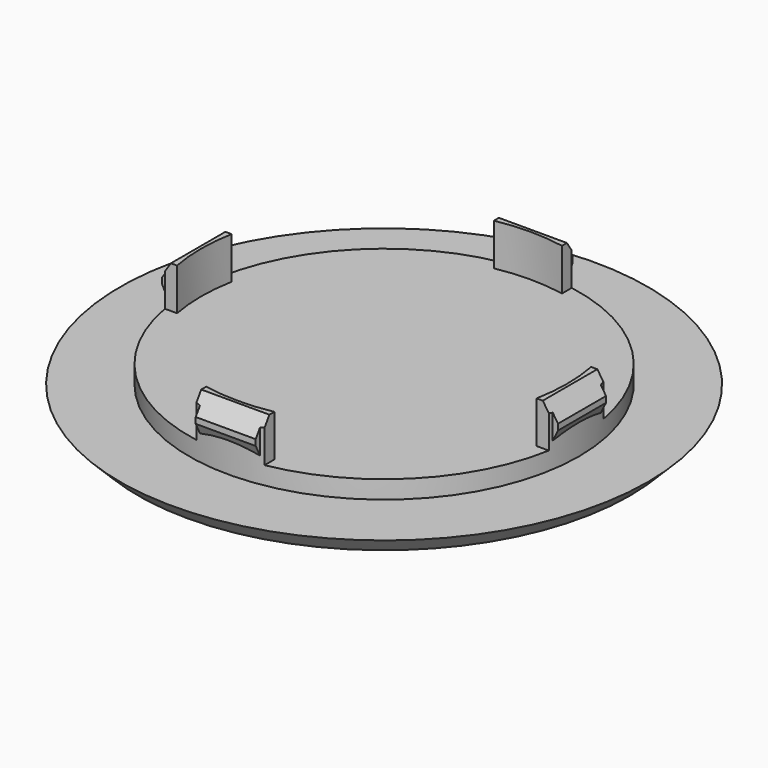
from build123d import *

# Parameters (mm, degrees)
F0_R          = 41
F1_DEPTH      = 3
F1_TAPER      = -45
F2_R          = 32.5
F3_DEPTH      = 10
F4_W          = 10
F4_H          = 6
F6_DEPTH      = 33
F6_DEPTH_BACK = 33
F7_W          = 10
F7_H          = 6
F8_DEPTH      = 33
F8_DEPTH_BACK = 33
F5_R          = 30.5
F9_DEPTH      = 7
F12_DEPTH     = 7
F13_SIZE2     = 2
F13_SIZE      = 3
F13_2_SIZE2   = 2
F13_2_SIZE    = 3
F14_SIZE2     = 3
F14_SIZE      = 2
F14_2_SIZE2   = 3
F14_2_SIZE    = 2
F15_T4_DEPTH  = 20.3593154951
F15_S5_R      = 32.5
F15_T6_DEPTH  = 12
F15_T10_DEPTH = 20.3593154951
F15_S11_R     = 32.5
F15_T12_DEPTH = 12
F16_T4_DEPTH  = 20.3593154951
F16_S5_R      = 32.5
F16_T6_DEPTH  = 12
F16_T10_DEPTH = 20.3593154951
F16_S11_R     = 32.5
F16_T12_DEPTH = 12


# Not quite as in the source:
# - a fillet or chamfer that OpenCascade refuses, or shapes differently, is made with other operations: its cross-section is extruded or revolved along the edge and cut away or added


with BuildPart() as f1:
    # F0 (on Top) → F1 (new body)
    with BuildSketch(Plane.XY):
        Circle(F0_R)
    extrude(amount=F1_DEPTH, taper=F1_TAPER)

    # F2 (on face) → F3 (join)
    with BuildSketch(Plane.XY.offset(3)):
        Circle(F2_R)
    extrude(amount=F3_DEPTH)

    # F4 (on Front) → F6 (join, two sides)
    with BuildSketch(Plane.XZ) as f6_sk:
        with Locations((0, 10)):
            Rectangle(F4_W, F4_H)
    extrude(amount=F6_DEPTH)
    extrude(f6_sk.sketch, amount=-F6_DEPTH_BACK)

    # F7 (on Right) → F8 (join, two sides)
    with BuildSketch(Plane.YZ) as f8_sk:
        with Locations((0, 10)):
            Rectangle(F7_W, F7_H)
    extrude(amount=F8_DEPTH)
    extrude(f8_sk.sketch, amount=-F8_DEPTH_BACK)

    # F5 (on face) → F9 (cut)
    with BuildSketch(Plane.XY.offset(13)):
        Circle(F5_R)
    extrude(amount=-F9_DEPTH, mode=Mode.SUBTRACT)

    # F11 (on face) → F12 (cut)
    with BuildSketch(Plane.XY.offset(13)):
        with BuildLine():
            ThreePointArc((-5.6789083458, 32), (-22.9809703886, 22.9809703886), (-32, 5.6789083458))
            Line((-32, 5.6789083458), (-29.9666481275, 5.6789083458))
            ThreePointArc((-29.9666481275, 5.6789083458), (-21.5667568262, 21.5667568262), (-5.6789083458, 29.9666481275))
            Line((-5.6789083458, 29.9666481275), (-5.6789083458, 32))
        make_face()
        with BuildLine():
            ThreePointArc((-5.6789083458, 29.9666481275), (-21.5667568262, 21.5667568262), (-29.9666481275, 5.6789083458))
            ThreePointArc((-29.9666481275, 5.6789083458), (-30.5, 0), (-29.9666481275, -5.6789083458))
            ThreePointArc((-29.9666481275, -5.6789083458), (-21.5667568262, -21.5667568262), (-5.6789083458, -29.9666481275))
            ThreePointArc((-5.6789083458, -29.9666481275), (0, -30.5), (5.6789083458, -29.9666481275))
            ThreePointArc((5.6789083458, -29.9666481275), (21.5667568262, -21.5667568262), (29.9666481275, -5.6789083458))
            ThreePointArc((29.9666481275, -5.6789083458), (30.3663692915, -2.8519495183), (30.5, 0))
            ThreePointArc((30.5, 0), (30.3663692915, 2.8519495183), (29.9666481275, 5.6789083458))
            ThreePointArc((29.9666481275, 5.6789083458), (21.5667568262, 21.5667568262), (5.6789083458, 29.9666481275))
            ThreePointArc((5.6789083458, 29.9666481275), (0, 30.5), (-5.6789083458, 29.9666481275))
        make_face()
        with BuildLine():
            Line((5.6789083458, 32), (5.6789083458, 29.9666481275))
            ThreePointArc((5.6789083458, 29.9666481275), (21.5667568262, 21.5667568262), (29.9666481275, 5.6789083458))
            Line((29.9666481275, 5.6789083458), (32, 5.6789083458))
            ThreePointArc((32, 5.6789083458), (22.9809703886, 22.9809703886), (5.6789083458, 32))
        make_face()
        with BuildLine():
            ThreePointArc((29.9666481275, -5.6789083458), (21.5667568262, -21.5667568262), (5.6789083458, -29.9666481275))
            Line((5.6789083458, -29.9666481275), (5.6789083458, -32))
            ThreePointArc((5.6789083458, -32), (22.9809703886, -22.9809703886), (32, -5.6789083458))
            Line((32, -5.6789083458), (29.9666481275, -5.6789083458))
        make_face()
        with BuildLine():
            ThreePointArc((-5.6789083458, -29.9666481275), (-21.5667568262, -21.5667568262), (-29.9666481275, -5.6789083458))
            Line((-29.9666481275, -5.6789083458), (-32, -5.6789083458))
            ThreePointArc((-32, -5.6789083458), (-22.9809703886, -22.9809703886), (-5.6789083458, -32))
            Line((-5.6789083458, -32), (-5.6789083458, -29.9666481275))
        make_face()
    extrude(amount=-F12_DEPTH, mode=Mode.SUBTRACT)

    # F13
    f13_edges = [f1.edges().sort_by_distance(p)[0] for p in [
        (0, 33, 13),
    ]]
    f13_side = f1.faces().sort_by_distance((0, 33, 10))[0]
    chamfer(f13_edges, length=F13_SIZE, length2=F13_SIZE2, reference=f13_side)

    # F13#2
    f13_2_edges = [f1.edges().sort_by_distance(p)[0] for p in [
        (33, 0, 13),
    ]]
    f13_2_side = f1.faces().sort_by_distance((33, 0, 10))[0]
    chamfer(f13_2_edges, length=F13_2_SIZE, length2=F13_2_SIZE2, reference=f13_2_side)

    # F14
    f14_edges = [f1.edges().sort_by_distance(p)[0] for p in [
        (0, -33, 13),
    ]]
    f14_side = f1.faces().sort_by_distance((0, -31.618427, 13))[0]
    chamfer(f14_edges, length=F14_SIZE, length2=F14_SIZE2, reference=f14_side)

    # F14#2
    f14_2_edges = [f1.edges().sort_by_distance(p)[0] for p in [
        (-33, 0, 13),
    ]]
    f14_2_side = f1.faces().sort_by_distance((-31.618427, 0, 13))[0]
    chamfer(f14_2_edges, length=F14_2_SIZE, length2=F14_2_SIZE2, reference=f14_2_side)

    # F15: chamfer of 1 x 2 on 2 edges, made by hand


with BuildPart() as f15_tool2:
    # F15_s3 → F15_t4 (new body)
    with BuildSketch(Plane.XZ.offset(10.1796577476)):
        Polygon((32, 7), (33, 9), (33, 7), align=None)
    extrude(amount=-F15_T4_DEPTH)

    # F15_s5 → F15_t6 (cut, symmetric)
    with BuildSketch(Plane.XY.offset(8)):
        Circle(F15_S5_R)
    extrude(amount=F15_T6_DEPTH, both=True, mode=Mode.SUBTRACT)


with BuildPart() as f1_1:
    add(f1.part)

    # F15_t1: cut F15_tool2
    add(f15_tool2.part, mode=Mode.SUBTRACT)


with BuildPart() as f15_tool8:
    # F15_s9 → F15_t10 (new body)
    with BuildSketch(Plane.YZ.offset(-10.1796577476)):
        Polygon((32, 7), (33, 9), (33, 7), align=None)
    extrude(amount=F15_T10_DEPTH)

    # F15_s11 → F15_t12 (cut, symmetric)
    with BuildSketch(Plane.XY.offset(8)):
        Circle(F15_S11_R)
    extrude(amount=F15_T12_DEPTH, both=True, mode=Mode.SUBTRACT)


with BuildPart() as f1_2:
    add(f1_1.part)

    # F15_t7: cut F15_tool8
    add(f15_tool8.part, mode=Mode.SUBTRACT)

    # F16: chamfer of 2 x 1 on 2 edges, made by hand


with BuildPart() as f16_tool2:
    # F16_s3 → F16_t4 (new body)
    with BuildSketch(Plane.YZ.offset(-10.1796577476)):
        Polygon((-33, 9), (-32, 7), (-33, 7), align=None)
    extrude(amount=F16_T4_DEPTH)

    # F16_s5 → F16_t6 (cut, symmetric)
    with BuildSketch(Plane.XY.offset(8)):
        Circle(F16_S5_R)
    extrude(amount=F16_T6_DEPTH, both=True, mode=Mode.SUBTRACT)


with BuildPart() as f1_3:
    add(f1_2.part)

    # F16_t1: cut F16_tool2
    add(f16_tool2.part, mode=Mode.SUBTRACT)


with BuildPart() as f16_tool8:
    # F16_s9 → F16_t10 (new body)
    with BuildSketch(Plane.XZ.offset(10.1796577476)):
        Polygon((-33, 9), (-32, 7), (-33, 7), align=None)
    extrude(amount=-F16_T10_DEPTH)

    # F16_s11 → F16_t12 (cut, symmetric)
    with BuildSketch(Plane.XY.offset(8)):
        Circle(F16_S11_R)
    extrude(amount=F16_T12_DEPTH, both=True, mode=Mode.SUBTRACT)


with BuildPart() as f1_4:
    add(f1_3.part)

    # F16_t7: cut F16_tool8
    add(f16_tool8.part, mode=Mode.SUBTRACT)


solid = f1_4.part
